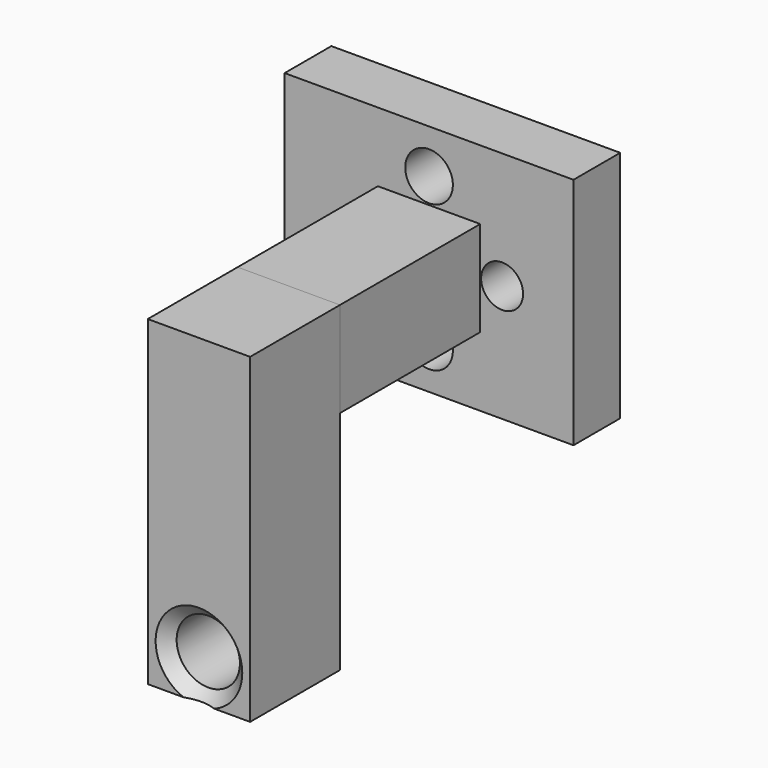
from build123d import *

# Parameters (mm, degrees)
F0_W     = 125.5568219279
F0_H     = 101.6
F0_R     = 9.122330494
F0_R_2   = 10.3539850451
F0_W_2   = 44.48986426
F0_H_2   = 41.3803607225
F1_DEPTH = 25.4
F2_DEPTH = 101.6
F3_W     = 44.48986426
F3_H     = 48.8234969616
F4_DEPTH = 139.7
F5_R     = 13.7554341803
F6_DEPTH = 150.4244969616


# Not quite as in the source:
# - a fillet or chamfer that OpenCascade refuses, or shapes differently, is made with other operations: its cross-section is extruded or revolved along the edge and cut away or added


with BuildPart() as f1:
    # F0 (on Front) → F1 (new body)
    with BuildSketch(Plane.XZ):
        Rectangle(F0_W, F0_H)
        with Locations((-31.75, 0)):
            Circle(F0_R, mode=Mode.SUBTRACT)
        with Locations((0, -31.75)):
            Circle(F0_R_2, mode=Mode.SUBTRACT)
        Rectangle(F0_W_2, F0_H_2, mode=Mode.SUBTRACT)
        with Locations((31.75, 0)):
            Circle(F0_R, mode=Mode.SUBTRACT)
        with Locations((0, 31.75)):
            Circle(F0_R_2, mode=Mode.SUBTRACT)
    extrude(amount=F1_DEPTH)

    # F0 (on Front) → F2 (join)
    with BuildSketch(Plane.XZ):
        Rectangle(F0_W_2, F0_H_2)
    extrude(amount=F2_DEPTH)


with BuildPart() as f4:
    # F3 (on face) → F4 (new body)
    with BuildSketch(Plane.XY.offset(20.6901803613)):
        with Locations((0, -126.0117484808)):
            Rectangle(F3_W, F3_H)
    extrude(amount=-F4_DEPTH)

    # F5 (on face) → F6 (cut, through all)
    with BuildSketch(Plane.XZ.offset(150.4234969616)):
        with Locations((0, -101.4029607177)):
            Circle(F5_R)
    extrude(amount=-F6_DEPTH, mode=Mode.SUBTRACT)

    # F7: chamfer of 5.08 on 3 edges, made by hand

    # F7_s1 → F7_t2 (revolve, cut)
    with BuildSketch(Plane.XY.offset(-101.4029607177)):
        Polygon((18.8354341803, -150.4234969616), (13.7554341803, -145.3434969616), (13.7554341803, -150.4234969616), align=None)
    revolve(axis=Axis((0, -150.4234969616, -101.4029607177), (0, -1, 0)), mode=Mode.SUBTRACT)

    # F7_s3 → F7_t4 (revolve, cut)
    with BuildSketch(Plane.XY.offset(-101.4029607177)):
        Polygon((18.8354341803, -101.6), (13.7554341803, -106.68), (13.7554341803, -101.6), align=None)
    revolve(axis=Axis((0, -101.6, -101.4029607177), (0, -1, 0)), mode=Mode.SUBTRACT)


solid = Compound([f1.part, f4.part])
